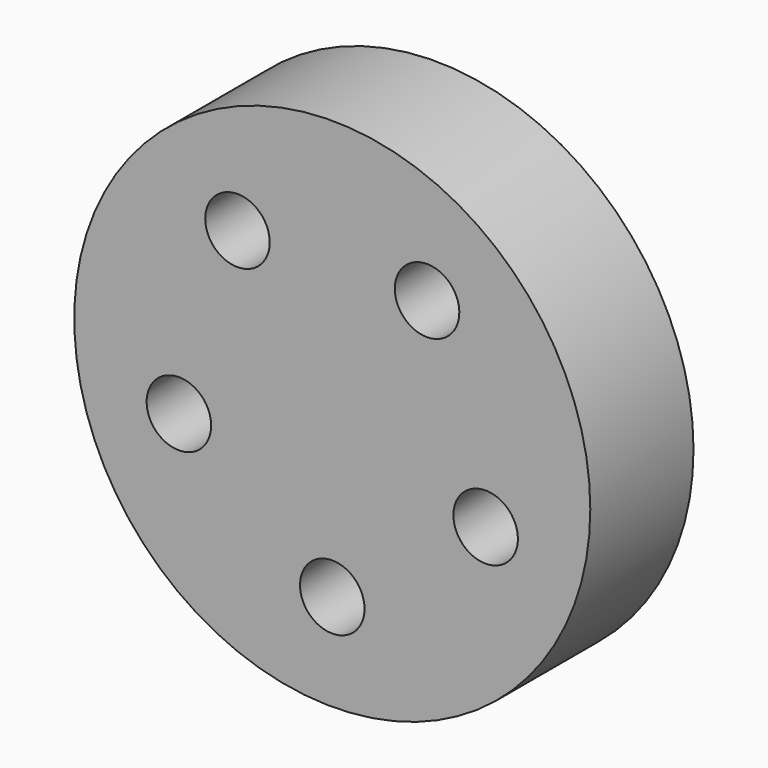
from build123d import *

# Parameters (mm, degrees)
F0_R            = 50.8
F1_DEPTH        = 25.4
F2_R            = 6.35
F3_DEPTH        = 25.4
F3_COPIES_COUNT = 5


# Not quite as in the source:
# - a pattern or mirror of a feature is missing from the dataset's text; its kind, count and spacing are read off the source's solid


with BuildPart() as f1:
    # F0 (on Front) → F1 (new body)
    with BuildSketch(Plane.XZ):
        Circle(F0_R)
    extrude(amount=F1_DEPTH)

    # F2 (on face) → F3 (cut)
    with BuildSketch(Plane.XZ.offset(25.4)):
        with Locations((0, -31.75)):
            Circle(F2_R)
    f3 = extrude(amount=-F3_DEPTH, mode=Mode.SUBTRACT)

    # F3_copies: F3 ×5 about axis
    f3_copies_axis = Axis((0, 0, 0), (0, 1, 0))
    for i in range(1, F3_COPIES_COUNT):
        add(f3.rotate(f3_copies_axis, i * 360 / F3_COPIES_COUNT), mode=Mode.SUBTRACT)


solid = f1.part
